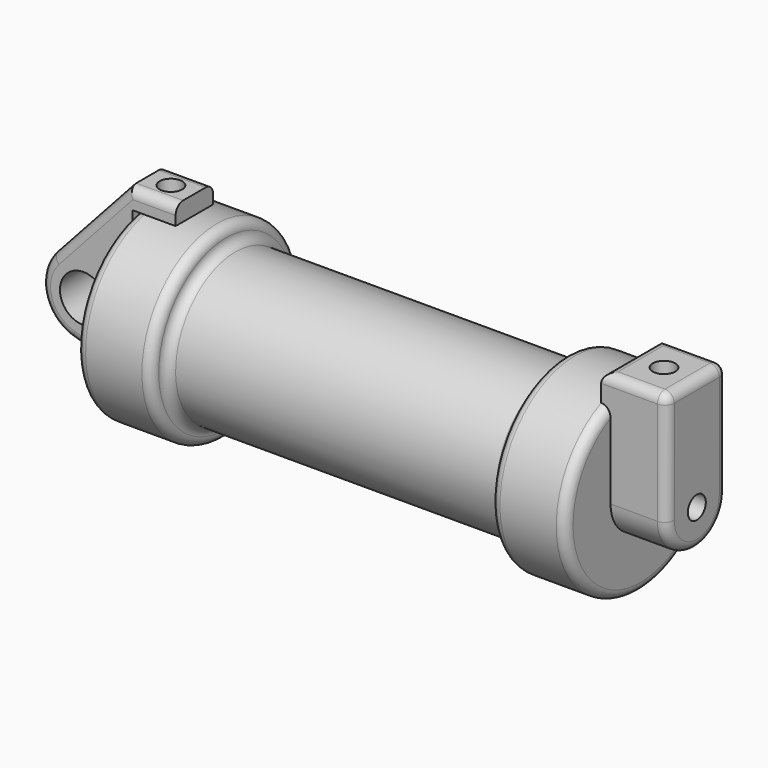
from build123d import *

# Parameters (mm, degrees)
F0_W          = 5.842
F0_H          = 12.7
F0_R          = 3.175
F2_DEPTH      = 3.175
F3_R          = 1.524
F4_DEPTH      = 7.62
F4_DEPTH_BACK = 1.27
F6_R          = 1.524
F7_DEPTH      = 17.78
F5_R          = 1.524
F8_DEPTH      = 10.414
F9_R          = 1.26999
F10_R         = 1.27
F11_R         = 1.27


# Not quite as in the source:
# - a fillet or chamfer is up to 0.001 mm smaller than in the source, because OpenCascade refuses the exact size


with BuildPart() as f1:
    # F0 (on Front) → F1 (revolve)
    with BuildSketch(Plane.XZ):
        with Locations((2.921, 6.35)):
            Rectangle(F0_W, F0_H)
        Polygon((5.842, 12.7), (5.842, 0), (66.294, 0), (66.294, 12.7), (56.134, 12.7), (56.134, 10.16), (10.16, 10.16), (10.16, 12.7), align=None)
    revolve(axis=Axis((33.147, 0, 0), (-1, 0, 0)))

    # F3 (on face) → F4 (join, two sides)
    with BuildSketch(Plane.YZ.offset(66.294)) as f4_sk:
        with BuildLine():
            ThreePointArc((-5.08, 0), (0, -5.08), (5.08, 0))
            ThreePointArc((5.08, 0), (0, 5.08), (-5.08, 0))
        make_face()
        Circle(F3_R, mode=Mode.SUBTRACT)
        with BuildLine():
            ThreePointArc((-5.08, 0), (0, 5.08), (5.08, 0))
            Line((5.08, 0), (5.08, 11.6397422652))
            ThreePointArc((5.08, 11.6397422652), (0, 12.7), (-5.08, 11.6397422652))
            Line((-5.08, 11.6397422652), (-5.08, 0))
        make_face()
        with BuildLine():
            ThreePointArc((-5.08, 11.6397422652), (0, 12.7), (5.08, 11.6397422652))
            Line((5.08, 11.6397422652), (5.08, 15.24))
            Line((5.08, 15.24), (-5.08, 15.24))
            Line((-5.08, 15.24), (-5.08, 11.6397422652))
        make_face()
    extrude(amount=F4_DEPTH)
    extrude(f4_sk.sketch, amount=-F4_DEPTH_BACK)

    # F5 (on face) → F8 (cut)
    with BuildSketch(Plane.XY.offset(15.24)):
        with Locations((69.469, 0)):
            Circle(F5_R)
    extrude(amount=-F8_DEPTH, mode=Mode.SUBTRACT)

    # F9 (radius 1.27 in the source; OpenCascade refuses exactly that, so slightly less here)
    f9_edges = [f1.edges().sort_by_distance(p)[0] for p in [
        (0, 0, -12.7),
        (10.16, 0, -12.7),
        (56.134, 0, -12.7),
        (66.294, 0, -12.7),
        (10.16, 0, -10.16),
        (56.134, 0, -10.16),
    ]]
    fillet(f9_edges, radius=F9_R)

    # F11
    f11_edges = [f1.edges().sort_by_distance(p)[0] for p in [
        (69.469, -5.08, 15.24),
        (73.914, 0, 15.24),
        (69.469, 5.08, 15.24),
        (73.914, 5.08, 7.62),
        (73.914, -5.08, 7.62),
        (65.024, 0, 15.24),
        (73.914, 0, -5.08),
    ]]
    fillet(f11_edges, radius=F11_R)


with BuildPart() as f2:
    # F0 (on Front) → F2 (new body, symmetric)
    with BuildSketch(Plane.XZ):
        with BuildLine():
            Line((-0.9398, 0), (0, 0))
            Line((0, 0), (0, 12.7))
            Line((0, 12.7), (5.842, 12.7))
            Line((5.842, 12.7), (5.842, 15.24))
            Line((5.842, 15.24), (-0.508, 15.24))
            Line((-0.508, 15.24), (-10.8806298187, 3.8475430269))
            ThreePointArc((-10.8806298187, 3.8475430269), (-4.5919612295, 5.3297205562), (-0.9398, 0))
        make_face()
        with BuildLine():
            ThreePointArc((-8.1826630726, -5.5069827884), (-3.1957909266, -4.5493385486), (-0.9398, 0))
            ThreePointArc((-0.9398, 0), (-4.5919612295, 5.3297205562), (-10.8806298187, 3.8475430269))
            ThreePointArc((-10.8806298187, 3.8475430269), (-12.1459778134, -1.5837270034), (-8.1826630726, -5.5069827884))
        make_face()
        with Locations((-6.6548, 0)):
            Circle(F0_R, mode=Mode.SUBTRACT)
        with BuildLine():
            Line((5.842, 0), (0, 0))
            Line((0, 0), (-0.9398, 0))
            ThreePointArc((-0.9398, 0), (-3.1957909266, -4.5493385486), (-8.1826630726, -5.5069827884))
            Line((-8.1826630726, -5.5069827884), (5.842, -9.398))
            Line((5.842, -9.398), (5.842, 0))
        make_face()
    extrude(amount=F2_DEPTH, both=True)

    # F6 (on face) → F7 (cut)
    with BuildSketch(Plane.XY.offset(15.24)):
        with Locations((2.667, 0)):
            Circle(F6_R)
    extrude(amount=-F7_DEPTH, mode=Mode.SUBTRACT)

    # F10
    f10_edges = [f2.edges().sort_by_distance(p)[0] for p in [
        (2.667, -3.175, 15.24),
        (-5.694315, -3.175, 9.543772),
        (2.667, 3.175, 15.24),
        (-5.694315, 3.175, 9.543772),
        (-12.145978, 3.175, -1.583727),
    ]]
    fillet(f10_edges, radius=F10_R)


solid = Compound([f1.part, f2.part])
